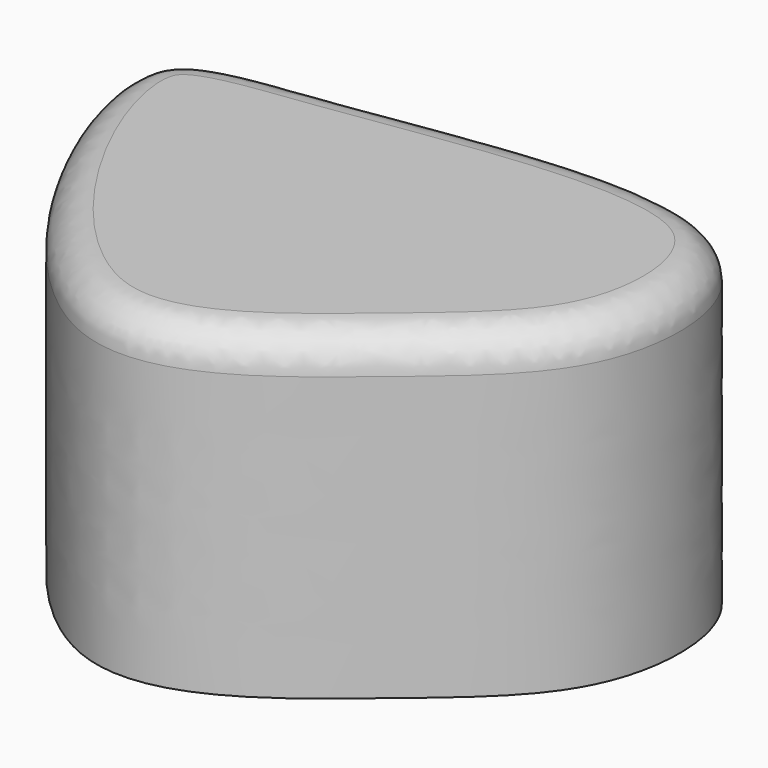
from build123d import *

# Parameters (mm, degrees)
F1_DEPTH = 43.52941
F2_R     = 5


with BuildPart() as f1:
    # F0 (on Top) → F1 (new body)
    with BuildSketch(Plane.XY):
        with BuildLine():
            add(Edge.make_bspline(
                [(-19.9331548065, 36.0762029886), (-2.9370422132, 38.3878699703), (36.6507331957, 46.7646188548), (39.1952668017, 10.7009418911), (19.9636348128, -4.724438126), (-14.1482745843, -34.2138204793), (-52.4994264417, 33.6699226101), (-31.3046000799, 34.5295555169), (-19.9331548065, 36.0762029886)],
                knots=[0, 0, 0, 0, 0.2046115804, 0.3423307865, 0.4872399184, 0.6540720636, 0.8631022608, 1, 1, 1, 1], degree=3))
        make_face()
    extrude(amount=F1_DEPTH)

    # F2
    f2_edges = [f1.edges().sort_by_distance(p)[0] for p in [
        (14.257232, -9.695925, 43.52941),
    ]]
    fillet(f2_edges, radius=F2_R)


solid = f1.part
